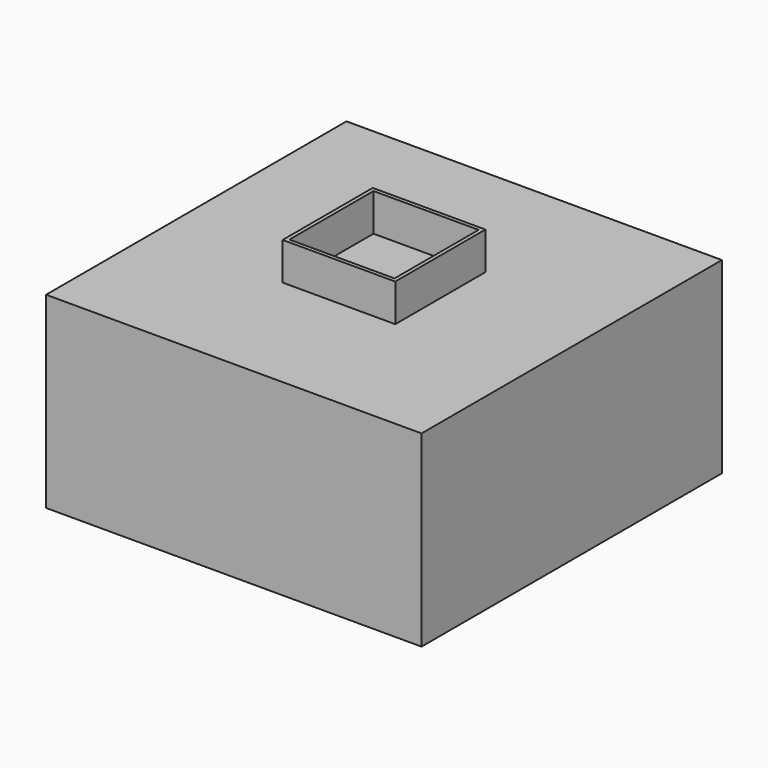
from build123d import *

# Parameters (mm, degrees)
F0_W     = 1000
F0_H     = 1000
F1_DEPTH = 500
F3_T     = -10
F2_W     = 300
F2_H     = 300
F4_DEPTH = 100
F5_T     = -10


# Not quite as in the source:
# - a shell that OpenCascade refuses in one call is made with other operations: the cavity is built on its own and cut out


with BuildPart() as f1:
    # F0 (on Top) → F1 (new body)
    with BuildSketch(Plane.XY):
        Rectangle(F0_W, F0_H)
    extrude(amount=F1_DEPTH)

    # F3
    f3_openings = [f1.faces().sort_by_distance(p)[0] for p in [
        (0, 0, 0),
    ]]
    offset(amount=F3_T, openings=f3_openings)

    # F2 (on face) → F4 (join)
    with BuildSketch(Plane.XY.offset(500)):
        Rectangle(F2_W, F2_H)
    extrude(amount=F4_DEPTH)

    # F5: a shell. OpenCascade refuses it in one call, so the cavity is built on its own and cut out:
    # the body offset inwards by the wall thickness, plus a prism from it out through each open face.
    f5_core = offset(f1.part, amount=F5_T, kind=Kind.INTERSECTION, mode=Mode.PRIVATE)
    f5_exits = [f5_core.faces().sort_by_distance(p)[0] for p in [
        (0, 0, 590),
    ]]
    add(f5_core, mode=Mode.SUBTRACT)
    extrude(f5_exits, amount=-F5_T, mode=Mode.SUBTRACT)


solid = f1.part
